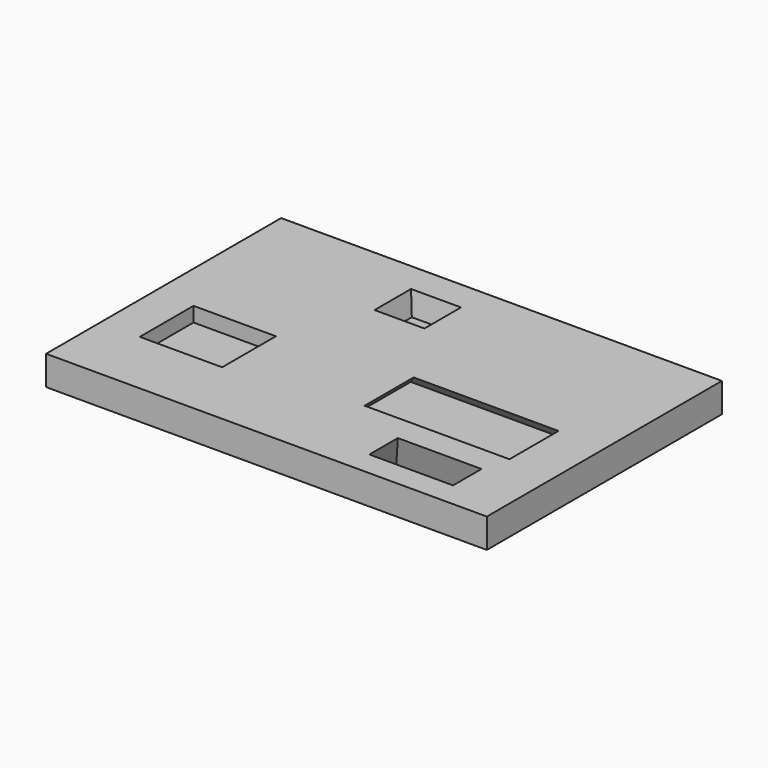
from build123d import *

# Parameters (mm, degrees)
F0_W      = 300
F0_H      = 200
F1_DEPTH  = 20
F2_W      = 56.0527034104
F2_H      = 45.7135215402
F3_DEPTH  = 10
F4_W      = 66.9058933854
F4_H      = 34.0227484703
F5_DEPTH  = 10
F6_W      = 98.600897938
F6_H      = 41.7043203488
F7_DEPTH  = 10
F7_TAPER  = -45
F8_W      = 32.641120255
F8_H      = 31.1660170555
F9_DEPTH  = 10
F9_TAPER  = -20
F10_W     = 33.9855737984
F10_H     = 31.0657545924
F11_DEPTH = 15
F11_TAPER = 10
F12_W     = 56.9754764438
F12_H     = 24.2112912238
F13_DEPTH = 25
F13_TAPER = -15


with BuildPart() as f1:
    # F0 (on Top) → F1 (new body)
    with BuildSketch(Plane.XY):
        with Locations((19.8950484647, 29.7908782959)):
            Rectangle(F0_W, F0_H)
    extrude(amount=F1_DEPTH)

    # F2 (on face) → F3 (cut)
    with BuildSketch(Plane.XY.offset(20)):
        with Locations((-75.3318350762, -1.0474342853)):
            Rectangle(F2_W, F2_H)
    extrude(amount=-F3_DEPTH, mode=Mode.SUBTRACT)

    # F4 (on face) → F5 (join)
    with BuildSketch(Plane.XY.offset(20)):
        with Locations((92.6642976701, 79.7481462359)):
            Rectangle(F4_W, F4_H)
    extrude(amount=-F5_DEPTH)

    # F6 (on face) → F7 (cut)
    with BuildSketch(Plane.XY.offset(20)):
        with Locations((88.7664388865, 9.6967569552)):
            Rectangle(F6_W, F6_H)
    extrude(amount=-F7_DEPTH, taper=F7_TAPER, mode=Mode.SUBTRACT)

    # F8 (on face) → F9 (join)
    with BuildSketch(Plane.XY.offset(20)):
        with Locations((-97.8116877377, 101.3978421688)):
            Rectangle(F8_W, F8_H)
    extrude(amount=-F9_DEPTH, taper=F9_TAPER)

    # F10 (on face) → F11 (cut)
    with BuildSketch(Plane.XY.offset(20)):
        with Locations((-8.2211010158, 93.6475135386)):
            Rectangle(F10_W, F10_H)
    extrude(amount=-F11_DEPTH, taper=F11_TAPER, mode=Mode.SUBTRACT)

    # F12 (on face) → F13 (cut)
    with BuildSketch(Plane.XY.offset(20)):
        with Locations((104.9904711545, -41.3090791553)):
            Rectangle(F12_W, F12_H)
    extrude(amount=-F13_DEPTH, taper=F13_TAPER, mode=Mode.SUBTRACT)


solid = f1.part
